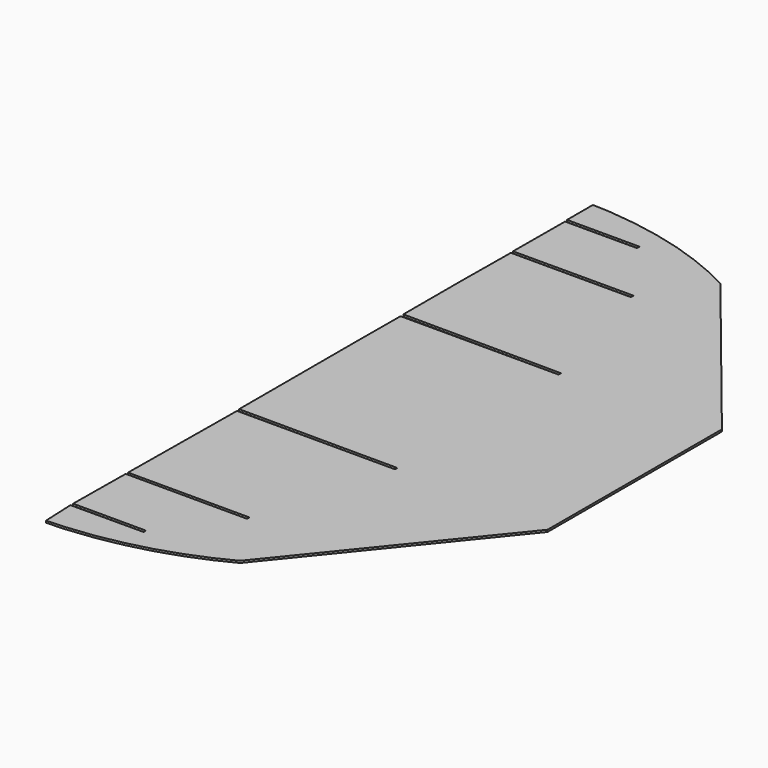
from build123d import *

# Parameters (mm, degrees)
F1_DEPTH = 1


# Not quite as in the source:
# - ends of sketch curves that miss each other by under 0.0002 mm in the source are joined


with BuildPart() as f1:
    # F0 (on Top) → F1 (new body)
    with BuildSketch(Plane.XY):
        Polygon((84.760502, 99.838331), (84.760502, 65.532372), (84.760502, 29.104707), (143.7776135408, 28.8903586668), (163.977411, 28.886699), (163.977411, 28.816993624), (164.3435, 28.815664), (164.3435, 27.535789), (163.977411, 27.535789), (163.977411, 27.386699), (85.0591829073, 27.400996887), (84.3979659422, -40.0634812645), (145.310694, -40.074967), (145.31063, -41.574967), (84.3837574867, -41.5131809608), (84.0646295035, -74.0740558181), (120.630506, -74.117418), (120.630358, -75.617418), (84.0482665226, -75.7435834112), (84.760502, -91.880651), (93.474501, -91.537649), (107.070486, -89.99767), (120.241516, -87.578631), (132.799484, -84.348639), (144.519505, -80.423663), (155.382483, -75.955654), (165.369519, -71.08065), (242.942492, 24.705363), (243.065503, 133.841338), (165.369519, 229.998345), (155.382483, 234.875351), (144.519505, 239.356344), (132.799484, 243.272341), (120.241516, 246.491352), (107.059515, 248.919369), (93.474501, 250.452351), (84.760502, 250.797334), (84.760502, 234.60194), (84.7707435172, 234.6018600186), (84.770746, 234.626524), (121.161056, 234.620025), (121.160905, 233.120025), (121.132491, 233.1200300745), (121.132491, 233.026024), (85.060504, 233.026024), (84.910536, 200.618297), (145.27452, 200.708488), (145.27452, 199.072799), (85.060504, 199.072799), (84.760502, 168.454341), (84.760502, 132.02771), (164.127413, 131.611891), (164.127413, 130.111891), (84.910503, 130.126243), (84.7605566, 99.8493557296), align=None)
    extrude(amount=F1_DEPTH)


solid = f1.part
